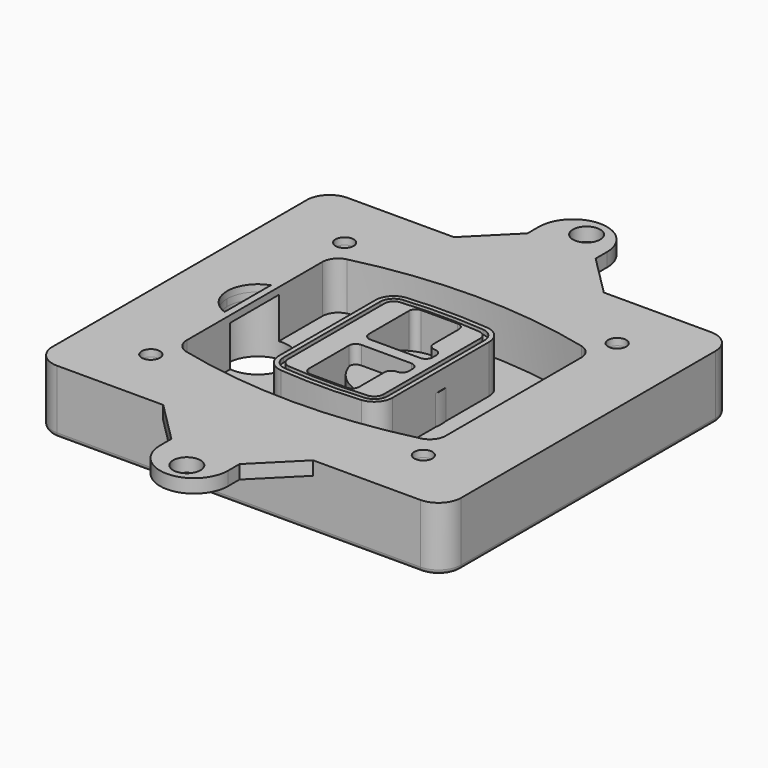
from build123d import *

# Parameters (mm, degrees)
F0_R      = 4
F1_DEPTH  = 25
F2_DEPTH  = 3
F3_DEPTH  = 18
F5_DEPTH  = 21
F6_DEPTH  = 2
F8_DEPTH  = 20
F9_DEPTH  = 16
F10_DEPTH = 25
F7_R      = 6
F7_R_2    = 4
F11_DEPTH = 6
F13_DEPTH = 9
F15_R     = 2
F16_R     = 6
F16_R_2   = 4
F17_DEPTH = 3


# Not quite as in the source:
# - a feature of the source that left no trace in its solid (it failed there, or was rolled back) is left out
# - a feature names something its author has since deleted; it is built from what else it names


with BuildPart() as f1:
    # F0 (on Top) → F1 (new body)
    with BuildSketch(Plane.XY):
        with BuildLine():
            ThreePointArc((-90, -70), (-87.0710678119, -77.0710678119), (-80, -80))
            Line((-80, -80), (80, -80))
            ThreePointArc((80, -80), (87.0710678119, -77.0710678119), (90, -70))
            Line((90, -70), (90, 70))
            ThreePointArc((90, 70), (87.0710678119, 77.0710678119), (80, 80))
            Line((80, 80), (-80, 80))
            ThreePointArc((-80, 80), (-87.0710678119, 77.0710678119), (-90, 70))
            Line((-90, 70), (-90, -70))
        make_face()
        with Locations((-60, -53.3333333333)):
            Circle(F0_R, mode=Mode.SUBTRACT)
        with Locations((60, -53.3333333333)):
            Circle(F0_R, mode=Mode.SUBTRACT)
        with Locations((-60, 53.3333333333)):
            Circle(F0_R, mode=Mode.SUBTRACT)
        with BuildLine():
            ThreePointArc((-64, 37.2990447398), (-61.0143011354, 45.9411029726), (-53.3306899286, 50.8970778549))
            ThreePointArc((-53.3306899286, 50.8970778549), (0, 57.3333333333), (53.3306899286, 50.8970778549))
            ThreePointArc((53.3306899286, 50.8970778549), (61.0143011354, 45.9411029726), (64, 37.2990447398))
            Line((64, 37.2990447398), (64, -37.2990447398))
            ThreePointArc((64, -37.2990447398), (61.0143011354, -45.9411029726), (53.3306899286, -50.8970778549))
            ThreePointArc((53.3306899286, -50.8970778549), (0, -57.3333333333), (-53.3306899286, -50.8970778549))
            ThreePointArc((-53.3306899286, -50.8970778549), (-61.0143011354, -45.9411029726), (-64, -37.2990447398))
            Line((-64, -37.2990447398), (-64, 37.2990447398))
        make_face(mode=Mode.SUBTRACT)
        with Locations((60, 53.3333333333)):
            Circle(F0_R, mode=Mode.SUBTRACT)
        with BuildLine():
            ThreePointArc((53.3306899286, 50.8970778549), (0, 57.3333333333), (-53.3306899286, 50.8970778549))
            ThreePointArc((-53.3306899286, 50.8970778549), (-61.0143011354, 45.9411029726), (-64, 37.2990447398))
            Line((-64, 37.2990447398), (-64, -37.2990447398))
            ThreePointArc((-64, -37.2990447398), (-61.0143011354, -45.9411029726), (-53.3306899286, -50.8970778549))
            ThreePointArc((-53.3306899286, -50.8970778549), (0, -57.3333333333), (53.3306899286, -50.8970778549))
            ThreePointArc((53.3306899286, -50.8970778549), (61.0143011354, -45.9411029726), (64, -37.2990447398))
            Line((64, -37.2990447398), (64, 37.2990447398))
            ThreePointArc((64, 37.2990447398), (61.0143011354, 45.9411029726), (53.3306899286, 50.8970778549))
        make_face()
        with BuildLine():
            Line((-60, -37.2990447398), (-60, 37.2990447398))
            ThreePointArc((-60, 37.2990447398), (-57.8673579538, 43.4719434775), (-52.3790642347, 47.0119255363))
            ThreePointArc((-52.3790642347, 47.0119255363), (0, 53.3333333333), (52.3790642347, 47.0119255363))
            ThreePointArc((52.3790642347, 47.0119255363), (57.8673579538, 43.4719434775), (60, 37.2990447398))
            Line((60, 37.2990447398), (60, -37.2990447398))
            ThreePointArc((60, -37.2990447398), (57.8673579538, -43.4719434775), (52.3790642347, -47.0119255363))
            ThreePointArc((52.3790642347, -47.0119255363), (0, -53.3333333333), (-52.3790642347, -47.0119255363))
            ThreePointArc((-52.3790642347, -47.0119255363), (-57.8673579538, -43.4719434775), (-60, -37.2990447398))
        make_face(mode=Mode.SUBTRACT)
        with BuildLine():
            ThreePointArc((-52.3790642347, 47.0119255363), (-57.8673579538, 43.4719434775), (-60, 37.2990447398))
            Line((-60, 37.2990447398), (-60, -37.2990447398))
            ThreePointArc((-60, -37.2990447398), (-57.8673579538, -43.4719434775), (-52.3790642347, -47.0119255363))
            ThreePointArc((-52.3790642347, -47.0119255363), (0, -53.3333333333), (52.3790642347, -47.0119255363))
            ThreePointArc((52.3790642347, -47.0119255363), (57.8673579538, -43.4719434775), (60, -37.2990447398))
            Line((60, -37.2990447398), (60, 37.2990447398))
            ThreePointArc((60, 37.2990447398), (57.8673579538, 43.4719434775), (52.3790642347, 47.0119255363))
            ThreePointArc((52.3790642347, 47.0119255363), (0, 53.3333333333), (-52.3790642347, 47.0119255363))
        make_face()
        with BuildLine():
            ThreePointArc((51.6653449643, 44.0980612973), (55.5071505677, 41.6200738562), (57, 37.2990447398))
            Line((57, 37.2990447398), (57, -37.2990447398))
            ThreePointArc((57, -37.2990447398), (55.5071505677, -41.6200738562), (51.6653449643, -44.0980612973))
            ThreePointArc((51.6653449643, -44.0980612973), (0, -50.3333333333), (-51.6653449643, -44.0980612973))
            ThreePointArc((-51.6653449643, -44.0980612973), (-55.5071505677, -41.6200738562), (-57, -37.2990447398))
            Line((-57, -37.2990447398), (-57, 37.2990447398))
            ThreePointArc((-57, 37.2990447398), (-55.5071505677, 41.6200738562), (-51.6653449643, 44.0980612973))
            ThreePointArc((-51.6653449643, 44.0980612973), (0, 50.3333333333), (51.6653449643, 44.0980612973))
        make_face(mode=Mode.SUBTRACT)
        with BuildLine():
            Line((57, -37.2990447398), (57, 37.2990447398))
            ThreePointArc((57, 37.2990447398), (55.5071505677, 41.6200738562), (51.6653449643, 44.0980612973))
            ThreePointArc((51.6653449643, 44.0980612973), (0, 50.3333333333), (-51.6653449643, 44.0980612973))
            ThreePointArc((-51.6653449643, 44.0980612973), (-55.5071505677, 41.6200738562), (-57, 37.2990447398))
            Line((-57, 37.2990447398), (-57, -37.2990447398))
            ThreePointArc((-57, -37.2990447398), (-55.5071505677, -41.6200738562), (-51.6653449643, -44.0980612973))
            ThreePointArc((-51.6653449643, -44.0980612973), (0, -50.3333333333), (51.6653449643, -44.0980612973))
            ThreePointArc((51.6653449643, -44.0980612973), (55.5071505677, -41.6200738562), (57, -37.2990447398))
        make_face()
    extrude(amount=-F1_DEPTH)

    # F0 (on Top) → F2 (join)
    with BuildSketch(Plane.XY):
        with BuildLine():
            ThreePointArc((-52.3790642347, 47.0119255363), (-57.8673579538, 43.4719434775), (-60, 37.2990447398))
            Line((-60, 37.2990447398), (-60, -37.2990447398))
            ThreePointArc((-60, -37.2990447398), (-57.8673579538, -43.4719434775), (-52.3790642347, -47.0119255363))
            ThreePointArc((-52.3790642347, -47.0119255363), (0, -53.3333333333), (52.3790642347, -47.0119255363))
            ThreePointArc((52.3790642347, -47.0119255363), (57.8673579538, -43.4719434775), (60, -37.2990447398))
            Line((60, -37.2990447398), (60, 37.2990447398))
            ThreePointArc((60, 37.2990447398), (57.8673579538, 43.4719434775), (52.3790642347, 47.0119255363))
            ThreePointArc((52.3790642347, 47.0119255363), (0, 53.3333333333), (-52.3790642347, 47.0119255363))
        make_face()
        with BuildLine():
            ThreePointArc((51.6653449643, 44.0980612973), (55.5071505677, 41.6200738562), (57, 37.2990447398))
            Line((57, 37.2990447398), (57, -37.2990447398))
            ThreePointArc((57, -37.2990447398), (55.5071505677, -41.6200738562), (51.6653449643, -44.0980612973))
            ThreePointArc((51.6653449643, -44.0980612973), (0, -50.3333333333), (-51.6653449643, -44.0980612973))
            ThreePointArc((-51.6653449643, -44.0980612973), (-55.5071505677, -41.6200738562), (-57, -37.2990447398))
            Line((-57, -37.2990447398), (-57, 37.2990447398))
            ThreePointArc((-57, 37.2990447398), (-55.5071505677, 41.6200738562), (-51.6653449643, 44.0980612973))
            ThreePointArc((-51.6653449643, 44.0980612973), (0, 50.3333333333), (51.6653449643, 44.0980612973))
        make_face(mode=Mode.SUBTRACT)
    extrude(amount=F2_DEPTH)

    # F0 (on Top) → F3 (cut)
    with BuildSketch(Plane.XY):
        with BuildLine():
            Line((57, -37.2990447398), (57, 37.2990447398))
            ThreePointArc((57, 37.2990447398), (55.5071505677, 41.6200738562), (51.6653449643, 44.0980612973))
            ThreePointArc((51.6653449643, 44.0980612973), (0, 50.3333333333), (-51.6653449643, 44.0980612973))
            ThreePointArc((-51.6653449643, 44.0980612973), (-55.5071505677, 41.6200738562), (-57, 37.2990447398))
            Line((-57, 37.2990447398), (-57, -37.2990447398))
            ThreePointArc((-57, -37.2990447398), (-55.5071505677, -41.6200738562), (-51.6653449643, -44.0980612973))
            ThreePointArc((-51.6653449643, -44.0980612973), (0, -50.3333333333), (51.6653449643, -44.0980612973))
            ThreePointArc((51.6653449643, -44.0980612973), (55.5071505677, -41.6200738562), (57, -37.2990447398))
        make_face()
    extrude(amount=-F3_DEPTH, mode=Mode.SUBTRACT)

    # F4 (on face) → F5 (join, through all)
    with BuildSketch(Plane.XY.offset(3)):
        with BuildLine():
            ThreePointArc((-25, -26.587695628), (-22.8992979869, -31.9912392117), (-17.7004291845, -34.5569740744))
            ThreePointArc((-17.7004291845, -34.5569740744), (0, -35.3333333333), (17.7004291845, -34.5569740744))
            ThreePointArc((17.7004291845, -34.5569740744), (22.8992979869, -31.9912392117), (25, -26.587695628))
            Line((25, -26.587695628), (25, 26.587695628))
            ThreePointArc((25, 26.587695628), (22.8992979869, 31.9912392117), (17.7004291845, 34.5569740744))
            ThreePointArc((17.7004291845, 34.5569740744), (0, 35.3333333333), (-17.7004291845, 34.5569740744))
            ThreePointArc((-17.7004291845, 34.5569740744), (-22.8992979869, 31.9912392117), (-25, 26.587695628))
            Line((-25, 26.587695628), (-25, -26.587695628))
        make_face()
        with BuildLine():
            ThreePointArc((17.5253218884, 32.5646544628), (21.4244734902, 30.6403533158), (23, 26.587695628))
            Line((23, 26.587695628), (23, -26.587695628))
            ThreePointArc((23, -26.587695628), (21.4244734902, -30.6403533158), (17.5253218884, -32.5646544628))
            ThreePointArc((17.5253218884, -32.5646544628), (0, -33.3333333333), (-17.5253218884, -32.5646544628))
            ThreePointArc((-17.5253218884, -32.5646544628), (-21.4244734902, -30.6403533158), (-23, -26.587695628))
            Line((-23, -26.587695628), (-23, 26.587695628))
            ThreePointArc((-23, 26.587695628), (-21.4244734902, 30.6403533158), (-17.5253218884, 32.5646544628))
            ThreePointArc((-17.5253218884, 32.5646544628), (0, 33.3333333333), (17.5253218884, 32.5646544628))
        make_face(mode=Mode.SUBTRACT)
        with BuildLine():
            Line((23, -26.587695628), (23, 26.587695628))
            ThreePointArc((23, 26.587695628), (21.4244734902, 30.6403533158), (17.5253218884, 32.5646544628))
            ThreePointArc((17.5253218884, 32.5646544628), (0, 33.3333333333), (-17.5253218884, 32.5646544628))
            ThreePointArc((-17.5253218884, 32.5646544628), (-21.4244734902, 30.6403533158), (-23, 26.587695628))
            Line((-23, 26.587695628), (-23, -26.587695628))
            ThreePointArc((-23, -26.587695628), (-21.4244734902, -30.6403533158), (-17.5253218884, -32.5646544628))
            ThreePointArc((-17.5253218884, -32.5646544628), (0, -33.3333333333), (17.5253218884, -32.5646544628))
            ThreePointArc((17.5253218884, -32.5646544628), (21.4244734902, -30.6403533158), (23, -26.587695628))
        make_face()
        with BuildLine():
            ThreePointArc((17.3502145923, 30.5723348512), (19.9496489934, 29.2894674198), (21, 26.587695628))
            Line((21, 26.587695628), (21, -26.587695628))
            ThreePointArc((21, -26.587695628), (19.9496489934, -29.2894674198), (17.3502145923, -30.5723348512))
            ThreePointArc((17.3502145923, -30.5723348512), (0, -31.3333333333), (-17.3502145923, -30.5723348512))
            ThreePointArc((-17.3502145923, -30.5723348512), (-19.9496489934, -29.2894674198), (-21, -26.587695628))
            Line((-21, -26.587695628), (-21, 26.587695628))
            ThreePointArc((-21, 26.587695628), (-19.9496489934, 29.2894674198), (-17.3502145923, 30.5723348512))
            ThreePointArc((-17.3502145923, 30.5723348512), (0, 31.3333333333), (17.3502145923, 30.5723348512))
        make_face(mode=Mode.SUBTRACT)
        with BuildLine():
            Line((21, -26.587695628), (21, 26.587695628))
            ThreePointArc((21, 26.587695628), (19.9496489934, 29.2894674198), (17.3502145923, 30.5723348512))
            ThreePointArc((17.3502145923, 30.5723348512), (0, 31.3333333333), (-17.3502145923, 30.5723348512))
            ThreePointArc((-17.3502145923, 30.5723348512), (-19.9496489934, 29.2894674198), (-21, 26.587695628))
            Line((-21, 26.587695628), (-21, -26.587695628))
            ThreePointArc((-21, -26.587695628), (-19.9496489934, -29.2894674198), (-17.3502145923, -30.5723348512))
            ThreePointArc((-17.3502145923, -30.5723348512), (0, -31.3333333333), (17.3502145923, -30.5723348512))
            ThreePointArc((17.3502145923, -30.5723348512), (19.9496489934, -29.2894674198), (21, -26.587695628))
        make_face()
        with BuildLine():
            Line((-8, -2.5), (14, -2.5))
            ThreePointArc((14, -2.5), (16.1213203436, -3.3786796564), (17, -5.5))
            Line((17, -5.5), (17, -7.5))
            ThreePointArc((17, -7.5), (16.1213203436, -9.6213203436), (14, -10.5))
            ThreePointArc((14, -10.5), (11.8786796564, -11.3786796564), (11, -13.5))
            Line((11, -13.5), (11, -27.5))
            ThreePointArc((11, -27.5), (10.1213203436, -29.6213203436), (8, -30.5))
            Line((8, -30.5), (-8, -30.5))
            ThreePointArc((-8, -30.5), (-10.1213203436, -29.6213203436), (-11, -27.5))
            Line((-11, -27.5), (-11, -5.5))
            ThreePointArc((-11, -5.5), (-10.1213203436, -3.3786796564), (-8, -2.5))
        make_face(mode=Mode.SUBTRACT)
        with BuildLine():
            ThreePointArc((-8, 2.5), (-10.1213203436, 3.3786796564), (-11, 5.5))
            Line((-11, 5.5), (-11, 27.5))
            ThreePointArc((-11, 27.5), (-10.1213203436, 29.6213203436), (-8, 30.5))
            Line((-8, 30.5), (8, 30.5))
            ThreePointArc((8, 30.5), (10.1213203436, 29.6213203436), (11, 27.5))
            Line((11, 27.5), (11, 13.5))
            ThreePointArc((11, 13.5), (11.8786796564, 11.3786796564), (14, 10.5))
            ThreePointArc((14, 10.5), (16.1213203436, 9.6213203436), (17, 7.5))
            Line((17, 7.5), (17, 5.5))
            ThreePointArc((17, 5.5), (16.1213203436, 3.3786796564), (14, 2.5))
            Line((14, 2.5), (-8, 2.5))
        make_face(mode=Mode.SUBTRACT)
    extrude(amount=-F5_DEPTH)

    # F4 (on face) → F6 (cut)
    with BuildSketch(Plane.XY.offset(3)):
        with BuildLine():
            Line((23, -26.587695628), (23, 26.587695628))
            ThreePointArc((23, 26.587695628), (21.4244734902, 30.6403533158), (17.5253218884, 32.5646544628))
            ThreePointArc((17.5253218884, 32.5646544628), (0, 33.3333333333), (-17.5253218884, 32.5646544628))
            ThreePointArc((-17.5253218884, 32.5646544628), (-21.4244734902, 30.6403533158), (-23, 26.587695628))
            Line((-23, 26.587695628), (-23, -26.587695628))
            ThreePointArc((-23, -26.587695628), (-21.4244734902, -30.6403533158), (-17.5253218884, -32.5646544628))
            ThreePointArc((-17.5253218884, -32.5646544628), (0, -33.3333333333), (17.5253218884, -32.5646544628))
            ThreePointArc((17.5253218884, -32.5646544628), (21.4244734902, -30.6403533158), (23, -26.587695628))
        make_face()
        with BuildLine():
            ThreePointArc((17.3502145923, 30.5723348512), (19.9496489934, 29.2894674198), (21, 26.587695628))
            Line((21, 26.587695628), (21, -26.587695628))
            ThreePointArc((21, -26.587695628), (19.9496489934, -29.2894674198), (17.3502145923, -30.5723348512))
            ThreePointArc((17.3502145923, -30.5723348512), (0, -31.3333333333), (-17.3502145923, -30.5723348512))
            ThreePointArc((-17.3502145923, -30.5723348512), (-19.9496489934, -29.2894674198), (-21, -26.587695628))
            Line((-21, -26.587695628), (-21, 26.587695628))
            ThreePointArc((-21, 26.587695628), (-19.9496489934, 29.2894674198), (-17.3502145923, 30.5723348512))
            ThreePointArc((-17.3502145923, 30.5723348512), (0, 31.3333333333), (17.3502145923, 30.5723348512))
        make_face(mode=Mode.SUBTRACT)
    extrude(amount=-F6_DEPTH, mode=Mode.SUBTRACT)

    # F7 (on face) → F8 (join)
    with BuildSketch(Plane(origin=(0, 0, -25), x_dir=(1, 0, 0), z_dir=(0, 0, -1))):
        with BuildLine():
            ThreePointArc((-6.71157564, 0), (6.7567035675, 13.4682792075), (20.224982775, 0))
            Line((20.224982775, 0), (25.224982775, 0))
            ThreePointArc((25.224982775, 0), (6.7567035675, 18.4682792075), (-11.71157564, 0))
            Line((-11.71157564, 0), (-6.71157564, 0))
        make_face()
        with BuildLine():
            Line((-6.71157564, 0), (20.224982775, 0))
            ThreePointArc((20.224982775, 0), (6.7567035675, 13.4682792075), (-6.71157564, 0))
        make_face()
        with BuildLine():
            ThreePointArc((-6.71157564, 0), (6.7567035675, -13.4682792075), (20.224982775, 0))
            Line((20.224982775, 0), (-6.71157564, 0))
        make_face()
        with BuildLine():
            Line((25.224982775, 0), (20.224982775, 0))
            ThreePointArc((20.224982775, 0), (6.7567035675, -13.4682792075), (-6.71157564, 0))
            Line((-6.71157564, 0), (-11.71157564, 0))
            ThreePointArc((-11.71157564, 0), (6.7567035675, -18.4682792075), (25.224982775, 0))
        make_face()
    extrude(amount=-F8_DEPTH)

    # F7 (on face) → F9 (cut)
    with BuildSketch(Plane(origin=(0, 0, -25), x_dir=(1, 0, 0), z_dir=(0, 0, -1))):
        with BuildLine():
            Line((-6.71157564, 0), (20.224982775, 0))
            ThreePointArc((20.224982775, 0), (6.7567035675, 13.4682792075), (-6.71157564, 0))
        make_face()
        with BuildLine():
            ThreePointArc((-6.71157564, 0), (6.7567035675, -13.4682792075), (20.224982775, 0))
            Line((20.224982775, 0), (-6.71157564, 0))
        make_face()
    extrude(amount=-F9_DEPTH, mode=Mode.SUBTRACT)

    # F7 (on face) → F10 (cut)
    with BuildSketch(Plane(origin=(0, 0, -25), x_dir=(1, 0, 0), z_dir=(0, 0, -1))):
        with BuildLine():
            Line((-69.0318229325, 0), (-42.0952645175, 0))
            ThreePointArc((-42.0952645175, 0), (-55.563543725, 13.4682792075), (-69.0318229325, 0))
        make_face()
        with BuildLine():
            ThreePointArc((-69.0318229325, 0), (-55.563543725, -13.4682792075), (-42.0952645175, 0))
            Line((-42.0952645175, 0), (-69.0318229325, 0))
        make_face()
    extrude(amount=-F10_DEPTH, mode=Mode.SUBTRACT)

    # F7 (on face) → F11 (cut)
    with BuildSketch(Plane(origin=(0, 0, -25), x_dir=(1, 0, 0), z_dir=(0, 0, -1))):
        with Locations((60, -53.3333333333)):
            Circle(F7_R)
        with Locations((60, -53.3333333333)):
            Circle(F7_R_2, mode=Mode.SUBTRACT)
        with Locations((-60, -53.3333333333)):
            Circle(F7_R)
        with Locations((-60, -53.3333333333)):
            Circle(F7_R_2, mode=Mode.SUBTRACT)
        with Locations((-60, 53.3333333333)):
            Circle(F7_R)
        with Locations((-60, 53.3333333333)):
            Circle(F7_R_2, mode=Mode.SUBTRACT)
        with Locations((60, 53.3333333333)):
            Circle(F7_R)
        with Locations((60, 53.3333333333)):
            Circle(F7_R_2, mode=Mode.SUBTRACT)
    extrude(amount=-F11_DEPTH, mode=Mode.SUBTRACT)

    # F12 (on face) → F13 (cut, through all)
    with BuildSketch(Plane(origin=(0, 0, -9), x_dir=(1, 0, 0), z_dir=(0, 0, -1))):
        with BuildLine():
            ThreePointArc((20.224982775, 0), (20.1663399806, 1.2554664788), (19.9909222755, 2.5))
            Line((19.9909222755, 2.5), (14, 2.5))
            ThreePointArc((14, 2.5), (16.1213203436, 3.3786796564), (17, 5.5))
            Line((17, 5.5), (17, 7.5))
            ThreePointArc((17, 7.5), (16.1213203436, 9.6213203436), (14, 10.5))
            ThreePointArc((14, 10.5), (12.1627255951, 11.1284134507), (11.0951631559, 12.750384826))
            ThreePointArc((11.0951631559, 12.750384826), (11.0476113807, 12.7664660322), (11, 12.7823698976))
            Line((11, 12.7823698976), (11, -12.7823698976))
            ThreePointArc((11, -12.7823698976), (11.0476113807, -12.7664660322), (11.0951631559, -12.750384826))
            ThreePointArc((11.0951631559, -12.750384826), (12.1627255951, -11.1284134507), (14, -10.5))
            ThreePointArc((14, -10.5), (16.1213203436, -9.6213203436), (17, -7.5))
            Line((17, -7.5), (17, -5.5))
            ThreePointArc((17, -5.5), (16.1213203436, -3.3786796564), (14, -2.5))
            Line((14, -2.5), (19.9909222755, -2.5))
            ThreePointArc((19.9909222755, -2.5), (20.1663399806, -1.2554664788), (20.224982775, 0))
        make_face()
    extrude(amount=F13_DEPTH, mode=Mode.SUBTRACT)

    # F15
    f15_edges = [f1.edges().sort_by_distance(p)[0] for p in [
        (0, -80, -25),
        (-87.071068, -77.071068, -25),
        (-90, 0, -25),
        (-87.071068, 77.071068, -25),
        (87.071068, -77.071068, -25),
        (0, 80, -25),
        (90, 0, -25),
        (87.071068, 77.071068, -25),
    ]]
    fillet(f15_edges, radius=F15_R)

    # F16 (on face) → F17 (join, symmetric)
    with BuildSketch(Plane.XY):
        with BuildLine():
            Line((-15.2164168358, 98), (-33.2164168358, 80))
            Line((-33.2164168358, 80), (32.7835831642, 80))
            Line((32.7835831642, 80), (14.7835831642, 98))
            Line((14.7835831642, 98), (14.7835831642, 104.25))
            ThreePointArc((14.7835831642, 104.25), (-0.2164168358, 119.25), (-15.2164168358, 104.25))
            Line((-15.2164168358, 104.25), (-15.2164168358, 98))
        make_face()
        with Locations((1.1958405546, 110)):
            Circle(F16_R, mode=Mode.SUBTRACT)
        with BuildLine():
            Line((-33.2164168358, 80), (-80, 80))
            ThreePointArc((-80, 80), (-87.0710678119, 77.0710678119), (-90, 70))
            Line((-90, 70), (-90, -70))
            ThreePointArc((-90, -70), (-87.0710678119, -77.0710678119), (-80, -80))
            Line((-80, -80), (-33.2164168358, -80))
            Line((-33.2164168358, -80), (32.7835831642, -80))
            Line((32.7835831642, -80), (80, -80))
            ThreePointArc((80, -80), (87.0710678119, -77.0710678119), (90, -70))
            Line((90, -70), (90, 70))
            ThreePointArc((90, 70), (87.0710678119, 77.0710678119), (80, 80))
            Line((80, 80), (32.7835831642, 80))
            Line((32.7835831642, 80), (-33.2164168358, 80))
        make_face()
        with Locations((-60, -53.3333333333)):
            Circle(F16_R_2, mode=Mode.SUBTRACT)
        with Locations((60, -53.3333333333)):
            Circle(F16_R_2, mode=Mode.SUBTRACT)
        with Locations((-60, 53.3333333333)):
            Circle(F16_R_2, mode=Mode.SUBTRACT)
        with BuildLine():
            Line((-60, 12.7166190685), (-60, 37.2990447398))
            ThreePointArc((-60, 37.2990447398), (-57.8673579538, 43.4719434775), (-52.3790642347, 47.0119255363))
            ThreePointArc((-52.3790642347, 47.0119255363), (0, 53.3333333333), (52.3790642347, 47.0119255363))
            ThreePointArc((52.3790642347, 47.0119255363), (57.8673579538, 43.4719434775), (60, 37.2990447398))
            Line((60, 37.2990447398), (60, -37.2990447398))
            ThreePointArc((60, -37.2990447398), (57.8673579538, -43.4719434775), (52.3790642347, -47.0119255363))
            ThreePointArc((52.3790642347, -47.0119255363), (0, -53.3333333333), (-52.3790642347, -47.0119255363))
            ThreePointArc((-52.3790642347, -47.0119255363), (-57.8673579538, -43.4719434775), (-60, -37.2990447398))
            Line((-60, -37.2990447398), (-60, -12.7166190685))
            ThreePointArc((-60, -12.7166190685), (-66.5441169481, -7.798817635), (-69.0318229325, 0))
            ThreePointArc((-69.0318229325, 0), (-66.5441169481, 7.798817635), (-60, 12.7166190685))
        make_face(mode=Mode.SUBTRACT)
        with Locations((60, 53.3333333333)):
            Circle(F16_R_2, mode=Mode.SUBTRACT)
        with BuildLine():
            Line((32.7835831642, -80), (-33.2164168358, -80))
            Line((-33.2164168358, -80), (-15.2164168358, -98))
            Line((-15.2164168358, -98), (-15.2164168358, -104.25))
            ThreePointArc((-15.2164168358, -104.25), (-0.2164168358, -119.25), (14.7835831642, -104.25))
            Line((14.7835831642, -104.25), (14.7835831642, -98))
            Line((14.7835831642, -98), (32.7835831642, -80))
        make_face()
        with Locations((1.1958405546, -110)):
            Circle(F16_R, mode=Mode.SUBTRACT)
    extrude(amount=F17_DEPTH, both=True)


solid = f1.part
